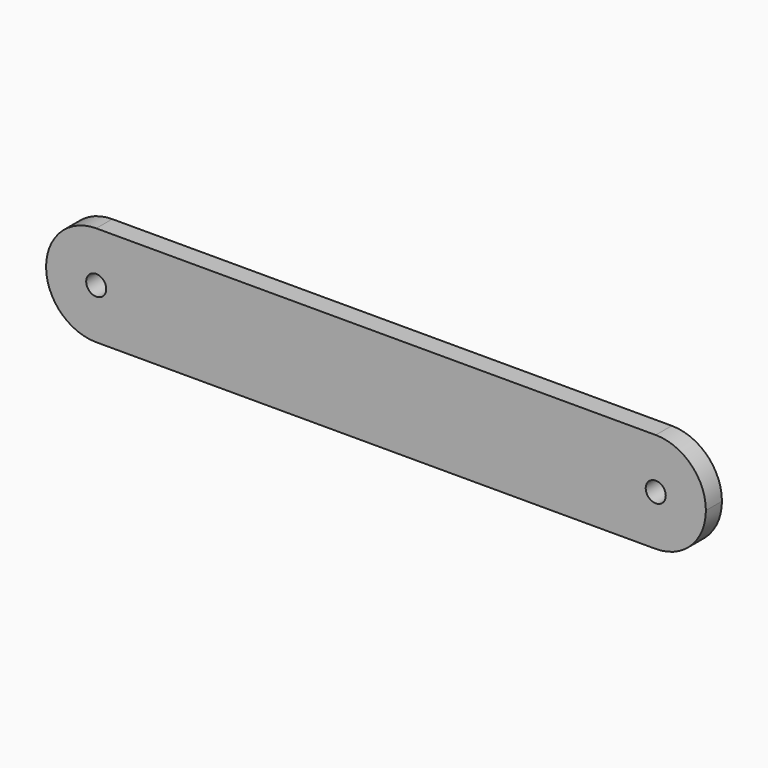
from build123d import *

# Parameters (mm, degrees)
F0_W     = 65.8
F0_H     = 10
F0_R     = 1
F1_DEPTH = 2
F2_R     = 4.99999


# Not quite as in the source:
# - a fillet or chamfer is up to 0.001 mm smaller than in the source, because OpenCascade refuses the exact size


with BuildPart() as f1:
    # F0 (on Front) → F1 (new body)
    with BuildSketch(Plane.XZ):
        with Locations((32.9, -5)):
            Rectangle(F0_W, F0_H)
        with Locations((5, -5)):
            Circle(F0_R, mode=Mode.SUBTRACT)
        with Locations((60.8, -5)):
            Circle(F0_R, mode=Mode.SUBTRACT)
    extrude(amount=F1_DEPTH)

    # F2 (radius 5 in the source; OpenCascade refuses exactly that, so slightly less here)
    f2_edges = [f1.edges().sort_by_distance(p)[0] for p in [
        (0, -1, 0),
        (0, -1, -10),
        (65.8, -1, 0),
        (65.8, -1, -10),
    ]]
    fillet(f2_edges, radius=F2_R)


solid = f1.part
